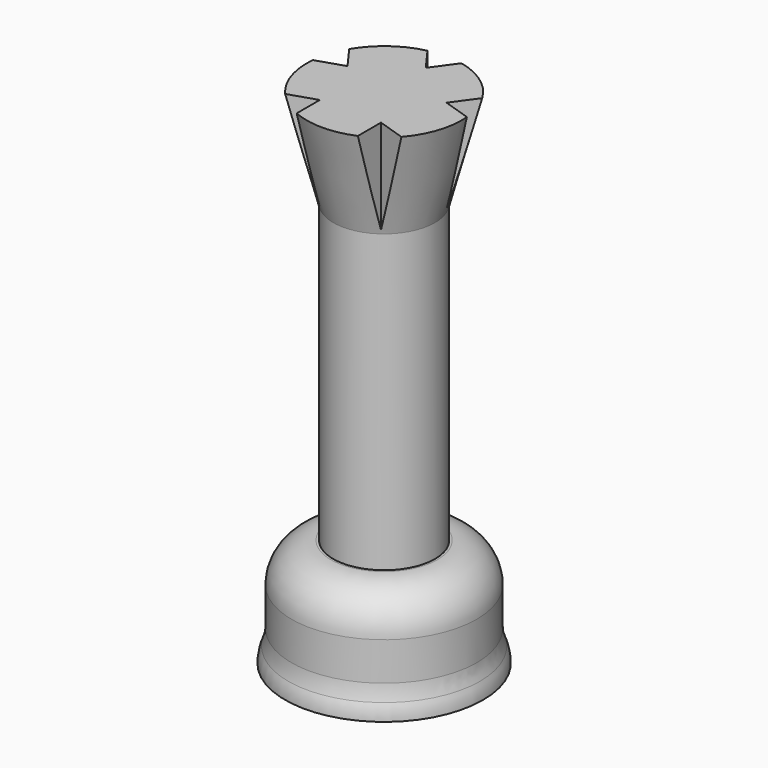
from build123d import *

# Parameters (mm, degrees)
F0_R      = 12.7368274584
F1_DEPTH  = 5.08
F2_R      = 5.07999
F3_R      = 11.9321398377
F4_DEPTH  = 13.97
F5_R      = 5.08
F6_R      = 6.5535099449
F7_DEPTH  = 24.13
F8_DEPTH  = 27.94
F8_FACE_R = 6.5535099449
F9_DEPTH  = 12.7
F9_TAPER  = -15
F11_DEPTH = 25.4


# Not quite as in the source:
# - a fillet or chamfer is up to 0.001 mm smaller than in the source, because OpenCascade refuses the exact size


with BuildPart() as f1:
    # F0 (on Top) → F1 (new body)
    with BuildSketch(Plane.XY):
        Circle(F0_R)
    extrude(amount=F1_DEPTH)

    # F2 (radius 5.08 in the source; OpenCascade refuses exactly that, so slightly less here)
    f2_edges = [f1.edges().sort_by_distance(p)[0] for p in [
        (-12.736827, 0, 5.08),
    ]]
    fillet(f2_edges, radius=F2_R)

    # F3 (on Top) → F4 (join)
    with BuildSketch(Plane.XY):
        Circle(F3_R)
    extrude(amount=F4_DEPTH)

    # F5
    f5_edges = [f1.edges().sort_by_distance(p)[0] for p in [
        (-11.93214, 0, 2.743746),
        (11.93214, 0, 8.356873),
        (-11.93214, 0, 13.97),
    ]]
    fillet(f5_edges, radius=F5_R)

    # F6 (on Top) → F7 (join)
    with BuildSketch(Plane.XY):
        Circle(F6_R)
    extrude(amount=F7_DEPTH)

    # F8 (add): a face of the model
    f8_faces = [f1.faces().sort_by_distance(p)[0] for p in [
        (0, 0, 24.13),
    ]]
    extrude(f8_faces, amount=F8_DEPTH)

    # F8_face (on face) → F9 (join)
    with BuildSketch(Plane.XY.offset(52.07)):
        Circle(F8_FACE_R)
    extrude(amount=F9_DEPTH, taper=F9_TAPER)

    # F10 (on face) → F11 (cut)
    with BuildSketch(Plane.XY.offset(64.77)):
        with BuildLine():
            Line((3.9382930845, -5.420595399), (3.9382930845, -9.1444538754))
            ThreePointArc((3.9382930845, -9.1444538754), (5.852263109, -8.0549491371), (7.4798929542, -6.5713309529))
            Line((7.4798929542, -6.5713309529), (3.9382930845, -5.420595399))
        make_face()
        with BuildLine():
            Line((8.5611211624, 5.0831479952), (6.3722920684, 2.0704832032))
            Line((6.3722920684, 2.0704832032), (9.9138919381, 0.9197476493))
            ThreePointArc((9.9138919381, 0.9197476493), (9.4691606215, 3.0767167927), (8.5611211624, 5.0831479952))
        make_face()
        with BuildLine():
            Line((-2.188829094, 9.7128891837), (0, 6.7002243917))
            Line((0, 6.7002243917), (2.188829094, 9.7128891837))
            ThreePointArc((2.188829094, 9.7128891837), (0, 9.9564646887), (-2.188829094, 9.7128891837))
        make_face()
        with BuildLine():
            ThreePointArc((-8.5611211624, 5.0831479952), (-9.4691606215, 3.0767167927), (-9.9138919381, 0.9197476493))
            Line((-9.9138919381, 0.9197476493), (-6.3722920684, 2.0704832032))
            Line((-6.3722920684, 2.0704832032), (-8.5611211624, 5.0831479952))
        make_face()
        with BuildLine():
            ThreePointArc((-7.4798929542, -6.5713309529), (-5.852263109, -8.0549491371), (-3.9382930845, -9.1444538754))
            Line((-3.9382930845, -9.1444538754), (-3.9382930845, -5.420595399))
            Line((-3.9382930845, -5.420595399), (-7.4798929542, -6.5713309529))
        make_face()
    extrude(amount=-F11_DEPTH, mode=Mode.SUBTRACT)


solid = f1.part
